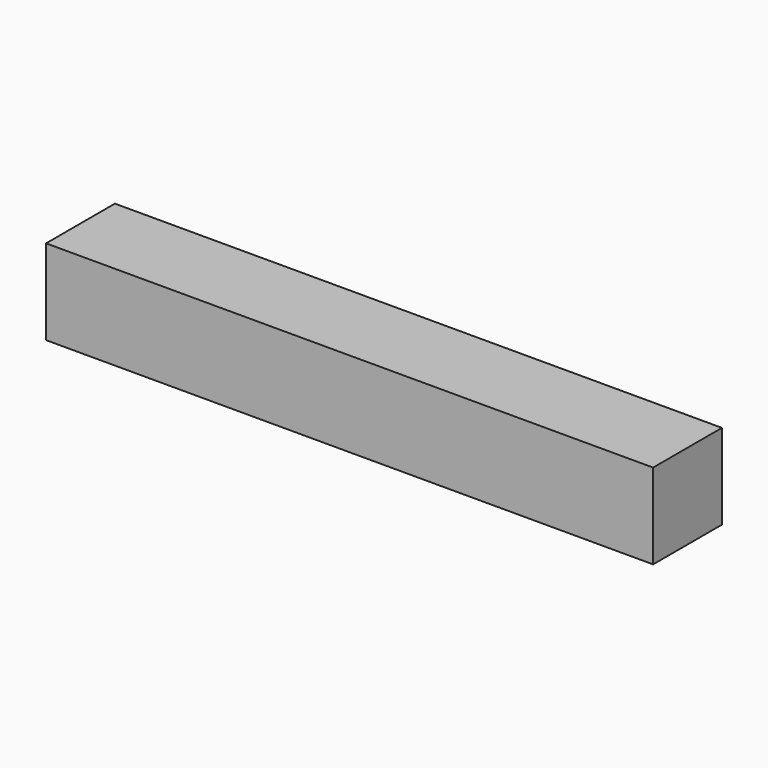
from build123d import *

# Parameters (mm, degrees)
F0_W     = 180.9011623263
F0_H     = 25.6362787914
F1_DEPTH = 25.4


# Not quite as in the source:
# - a feature of the source that left no trace in its solid (it failed there, or was rolled back) is left out


with BuildPart() as f1:
    # F0 (on Top) → F1 (new body)
    with BuildSketch(Plane.XY):
        with Locations((32.8723229468, 10.7506975764)):
            Rectangle(F0_W, F0_H)
    extrude(amount=F1_DEPTH)


solid = f1.part
